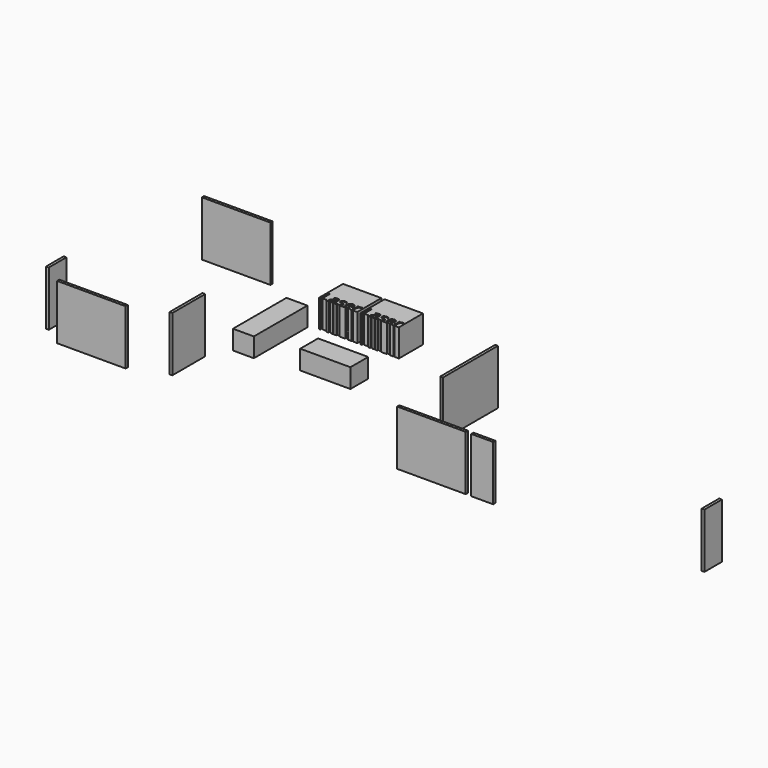
from build123d import *

# Parameters (mm, degrees)
F0_W     = 2479.91771698
F0_H     = 100
F0_W_2   = 20.08228302
F1_DEPTH = 2000
F0_W_3   = 100
F0_H_2   = 800
F0_W_4   = 2500
F0_W_5   = 800
F0_H_3   = 1500
F0_H_4   = 2500
F0_W_6   = 1828.8
F0_H_5   = 812.8
F4_DEPTH = 700
F0_W_7   = 762
F0_H_6   = 2438.4
F5_DEPTH = 1000


# Not quite as in the source:
# - the program builds the solid bodies; features that only make, move or delete a surface that nothing else refers to are left out


with BuildPart() as f1:
    # F0 (on Top) → F1 (new body)
    with BuildSketch(Plane.XY):
        with Locations((-9960.04114151, 3300)):
            Rectangle(F0_W, F0_H)
        with Locations((-8710.04114151, 3300)):
            Rectangle(F0_W_2, F0_H)
    extrude(amount=F1_DEPTH)


with BuildPart() as f1b:
    # F0 (on Top) → F1, piece 2 (new body)
    with BuildSketch(Plane.XY):
        with Locations((-11950, -2450)):
            Rectangle(F0_W_3, F0_H_2)
    extrude(amount=F1_DEPTH)


with BuildPart() as f1c:
    # F0 (on Top) → F1, piece 3 (new body)
    with BuildSketch(Plane.XY):
        with Locations((-9950, -3300)):
            Rectangle(F0_W_4, F0_H)
    extrude(amount=F1_DEPTH)


with BuildPart() as f1d:
    # F0 (on Top) → F1, piece 4 (new body)
    with BuildSketch(Plane.XY):
        with Locations((4300, -3300)):
            Rectangle(F0_W_5, F0_H)
    extrude(amount=F1_DEPTH)


with BuildPart() as f1e:
    # F0 (on Top) → F1, piece 5 (new body)
    with BuildSketch(Plane.XY):
        with Locations((2450, -3300)):
            Rectangle(F0_W_4, F0_H)
    extrude(amount=F1_DEPTH)


with BuildPart() as f1f:
    # F0 (on Top) → F1, piece 6 (new body)
    with BuildSketch(Plane.XY):
        with Locations((11950, -2450)):
            Rectangle(F0_W_3, F0_H_2)
    extrude(amount=F1_DEPTH)


with BuildPart() as f1g:
    # F0 (on Top) → F1, piece 7 (new body)
    with BuildSketch(Plane.XY):
        with Locations((-7450, -2100)):
            Rectangle(F0_W_3, F0_H_3)
    extrude(amount=F1_DEPTH)


with BuildPart() as f1h:
    # F0 (on Top) → F1, piece 8 (new body)
    with BuildSketch(Plane.XY):
        with Locations((1050, 115.6229972839)):
            Rectangle(F0_W_3, F0_H_4)
    extrude(amount=F1_DEPTH)


with BuildPart() as f4:
    # F0 (on Top) → F4 (new body)
    with BuildSketch(Plane.XY):
        with Locations((-3828.3553308487, 67.7179724663)):
            Rectangle(F0_W_6, F0_H_5)
    extrude(amount=F4_DEPTH)


with BuildPart() as f4b:
    # F0 (on Top) → F4, piece 2 (new body)
    with BuildSketch(Plane.XY):
        with Locations((-6626.9812164307, 645.5204336166)):
            Rectangle(F0_W_7, F0_H_6)
    extrude(amount=F4_DEPTH)


with BuildPart() as f5:
    # F0 (on Top) → F5 (new body)
    with BuildSketch(Plane.XY):
        with BuildLine():
            Line((-4528.5587310791, 3091.9769287109), (-5928.5587310791, 3091.9769287109))
            Line((-5928.5587310791, 3091.9769287109), (-5928.5587310791, 1991.9769287109))
            Line((-5928.5587310791, 1991.9769287109), (-5875.150882701, 1991.9769287109))
            Line((-5875.150882701, 1991.9769287109), (-5875.150882701, 2380.5445389649))
            Line((-5875.150882701, 2380.5445389649), (-5829.9923357444, 2380.5445389649))
            Line((-5829.9923357444, 2380.5445389649), (-5829.9923357444, 2032.88325844))
            Line((-5829.9923357444, 2032.88325844), (-5658.5429371294, 2032.88325844))
            Line((-5658.5429371294, 2032.88325844), (-5658.5429371294, 1991.9769287109))
            Line((-5658.5429371294, 1991.9769287109), (-5566.4860231589, 1991.9769287109))
            add(Edge.make_bspline(
                [(-5566.4860231589, 1991.9769287109), (-5583.9119205595, 1997.5660964187), (-5596.4605656071, 2008.9857976212)],
                knots=[0.4894320446, 0.4894320446, 0.4894320446, 1, 1, 1], degree=2))
            add(Edge.make_bspline(
                [(-5596.4605656071, 2008.9857976212), (-5621.0383811824, 2031.3524602381), (-5621.0383811824, 2072.5139230008)],
                knots=[0, 0, 0, 1, 1, 1], degree=2))
            add(Edge.make_bspline(
                [(-5621.0383811824, 2072.5139230008), (-5621.0383811824, 2160.7049083003), (-5479.9498135721, 2164.9571255278)],
                knots=[0, 0, 0, 1, 1, 1], degree=2))
            Line((-5479.9498135721, 2164.9571255278), (-5430.5390493879, 2166.5729680743))
            Line((-5430.5390493879, 2166.5729680743), (-5430.5390493879, 2184.6874134637))
            add(Edge.make_bspline(
                [(-5430.5390493879, 2184.6874134637), (-5430.5390493879, 2218.9602843178), (-5445.2517209953, 2235.2887984716)],
                knots=[0, 0, 0, 1, 1, 1], degree=2))
            add(Edge.make_bspline(
                [(-5445.2517209953, 2235.2887984716), (-5459.9643926026, 2251.6173126254), (-5492.4513322211, 2251.6173126254)],
                knots=[0, 0, 0, 1, 1, 1], degree=2))
            add(Edge.make_bspline(
                [(-5492.4513322211, 2251.6173126254), (-5528.850311689, 2251.6173126254), (-5574.7742577466, 2229.335694353)],
                knots=[0, 0, 0, 1, 1, 1], degree=2))
            Line((-5574.7742577466, 2229.335694353), (-5588.3813528748, 2263.0982991398))
            add(Edge.make_bspline(
                [(-5588.3813528748, 2263.0982991398), (-5566.8651337033, 2274.7493743433), (-5541.2242638212, 2281.3828332183)],
                knots=[0, 0, 0, 1, 1, 1], degree=2))
            add(Edge.make_bspline(
                [(-5541.2242638212, 2281.3828332183), (-5515.583393939, 2288.0162920933), (-5489.7299131955, 2288.0162920933)],
                knots=[0, 0, 0, 1, 1, 1], degree=2))
            add(Edge.make_bspline(
                [(-5489.7299131955, 2288.0162920933), (-5437.6827743302, 2288.0162920933), (-5412.5521705154, 2264.9267525477)],
                knots=[0, 0, 0, 1, 1, 1], degree=2))
            add(Edge.make_bspline(
                [(-5412.5521705154, 2264.9267525477), (-5387.4215667005, 2241.837213002), (-5387.4215667005, 2190.8106062714)],
                knots=[0, 0, 0, 1, 1, 1], degree=2))
            Line((-5387.4215667005, 2190.8106062714), (-5387.4215667005, 1991.9769287109))
            Line((-5387.4215667005, 1991.9769287109), (-5279.165564816, 1991.9769287109))
            add(Edge.make_bspline(
                [(-5279.165564816, 1991.9769287109), (-5299.4656029078, 1996.5398412124), (-5314.3684747311, 2004.9887134273)],
                knots=[0.5400617249, 0.5400617249, 0.5400617249, 1, 1, 1], degree=2))
            Line((-5314.3684747311, 2004.9887134273), (-5314.3684747311, 2045.8950431563))
            add(Edge.make_bspline(
                [(-5314.3684747311, 2045.8950431563), (-5293.362521627, 2035.2645000874), (-5269.3374942913, 2029.183829452)],
                knots=[0, 0, 0, 1, 1, 1], degree=2))
            add(Edge.make_bspline(
                [(-5269.3374942913, 2029.183829452), (-5245.3124669557, 2023.1031588166), (-5222.9458043387, 2023.1031588166)],
                knots=[0, 0, 0, 1, 1, 1], degree=2))
            add(Edge.make_bspline(
                [(-5222.9458043387, 2023.1031588166), (-5188.417800451, 2023.1031588166), (-5169.8356111666, 2034.116401436)],
                knots=[0, 0, 0, 1, 1, 1], degree=2))
            add(Edge.make_bspline(
                [(-5169.8356111666, 2034.116401436), (-5151.2534218822, 2045.1296440554), (-5151.2534218822, 2067.751439706)],
                knots=[0, 0, 0, 1, 1, 1], degree=2))
            add(Edge.make_bspline(
                [(-5151.2534218822, 2067.751439706), (-5151.2534218822, 2084.7603086162), (-5165.9660934895, 2096.8366055424)],
                knots=[0, 0, 0, 1, 1, 1], degree=2))
            add(Edge.make_bspline(
                [(-5165.9660934895, 2096.8366055424), (-5180.6787650968, 2108.9129024687), (-5223.5411147506, 2125.4115053116)],
                knots=[0, 0, 0, 1, 1, 1], degree=2))
            add(Edge.make_bspline(
                [(-5223.5411147506, 2125.4115053116), (-5264.192311446, 2140.5493986417), (-5281.3287468731, 2151.860296467)],
                knots=[0, 0, 0, 1, 1, 1], degree=2))
            add(Edge.make_bspline(
                [(-5281.3287468731, 2151.860296467), (-5298.4651823001, 2163.1711942923), (-5306.8420502384, 2177.5011663491)],
                knots=[0, 0, 0, 1, 1, 1], degree=2))
            add(Edge.make_bspline(
                [(-5306.8420502384, 2177.5011663491), (-5315.2189181767, 2191.831138406), (-5315.2189181767, 2211.7315150309)],
                knots=[0, 0, 0, 1, 1, 1], degree=2))
            add(Edge.make_bspline(
                [(-5315.2189181767, 2211.7315150309), (-5315.2189181767, 2247.3650953979), (-5286.2187966847, 2267.9883489515)],
                knots=[0, 0, 0, 1, 1, 1], degree=2))
            add(Edge.make_bspline(
                [(-5286.2187966847, 2267.9883489515), (-5257.2186751928, 2288.6116025051), (-5206.787378874, 2288.6116025051)],
                knots=[0, 0, 0, 1, 1, 1], degree=2))
            add(Edge.make_bspline(
                [(-5206.787378874, 2288.6116025051), (-5159.7578563373, 2288.6116025051), (-5114.7693980697, 2269.4766249811)],
                knots=[0, 0, 0, 1, 1, 1], degree=2))
            Line((-5114.7693980697, 2269.4766249811), (-5130.5026018117, 2233.5879115806))
            add(Edge.make_bspline(
                [(-5130.5026018117, 2233.5879115806), (-5174.3004392555, 2251.6173126254), (-5209.9340196224, 2251.6173126254)],
                knots=[0, 0, 0, 1, 1, 1], degree=2))
            add(Edge.make_bspline(
                [(-5209.9340196224, 2251.6173126254), (-5241.3153827618, 2251.6173126254), (-5257.2611973651, 2241.7946908298)],
                knots=[0, 0, 0, 1, 1, 1], degree=2))
            add(Edge.make_bspline(
                [(-5257.2611973651, 2241.7946908298), (-5273.2070119684, 2231.9720690341), (-5273.2070119684, 2214.7080670902)],
                knots=[0, 0, 0, 1, 1, 1], degree=2))
            add(Edge.make_bspline(
                [(-5273.2070119684, 2214.7080670902), (-5273.2070119684, 2202.9719475422), (-5267.2113856776, 2194.765168293)],
                knots=[0, 0, 0, 1, 1, 1], degree=2))
            add(Edge.make_bspline(
                [(-5267.2113856776, 2194.765168293), (-5261.2157593867, 2186.5583890438), (-5247.9488416367, 2179.1170088956)],
                knots=[0, 0, 0, 1, 1, 1], degree=2))
            add(Edge.make_bspline(
                [(-5247.9488416367, 2179.1170088956), (-5234.6819238868, 2171.6756287474), (-5196.9222349061, 2157.5582675519)],
                knots=[0, 0, 0, 1, 1, 1], degree=2))
            add(Edge.make_bspline(
                [(-5196.9222349061, 2157.5582675519), (-5145.1302290745, 2138.6784230616), (-5126.9307393406, 2119.5434455376)],
                knots=[0, 0, 0, 1, 1, 1], degree=2))
            add(Edge.make_bspline(
                [(-5126.9307393406, 2119.5434455376), (-5108.7312496066, 2100.4084680136), (-5108.7312496066, 2071.4083465217)],
                knots=[0, 0, 0, 1, 1, 1], degree=2))
            add(Edge.make_bspline(
                [(-5108.7312496066, 2071.4083465217), (-5108.7312496066, 2030.7571498262), (-5139.0070362668, 2008.6881424152)],
                knots=[0, 0, 0, 1, 1, 1], degree=2))
            add(Edge.make_bspline(
                [(-5139.0070362668, 2008.6881424152), (-5154.3652891477, 1997.4930114529), (-5176.0263007473, 1991.9769287109)],
                knots=[0, 0, 0, 0.5072784088, 0.5072784088, 0.5072784088], degree=2))
            Line((-5176.0263007473, 1991.9769287109), (-4957.8182645501, 1991.9769287109))
            add(Edge.make_bspline(
                [(-4957.8182645501, 1991.9769287109), (-4992.2307684042, 2001.143802815), (-5015.8203031846, 2025.9946665314)],
                knots=[0.3688754729, 0.3688754729, 0.3688754729, 1, 1, 1], degree=2))
            add(Edge.make_bspline(
                [(-5015.8203031846, 2025.9946665314), (-5053.1972926148, 2065.3701980585), (-5053.1972926148, 2135.191604935)],
                knots=[0, 0, 0, 1, 1, 1], degree=2))
            add(Edge.make_bspline(
                [(-5053.1972926148, 2135.191604935), (-5053.1972926148, 2205.6933665678), (-5018.4992000379, 2247.1524845365)],
                knots=[0, 0, 0, 1, 1, 1], degree=2))
            add(Edge.make_bspline(
                [(-5018.4992000379, 2247.1524845365), (-4983.8011074611, 2288.6116025051), (-4925.2905984099, 2288.6116025051)],
                knots=[0, 0, 0, 1, 1, 1], degree=2))
            add(Edge.make_bspline(
                [(-4925.2905984099, 2288.6116025051), (-4870.6070848636, 2288.6116025051), (-4838.7154556569, 2252.5953225877)],
                knots=[0, 0, 0, 1, 1, 1], degree=2))
            add(Edge.make_bspline(
                [(-4838.7154556569, 2252.5953225877), (-4806.8238264503, 2216.5790426704), (-4806.8238264503, 2157.5582675519)],
                knots=[0, 0, 0, 1, 1, 1], degree=2))
            Line((-4806.8238264503, 2157.5582675519), (-4806.8238264503, 2129.6637225391))
            Line((-4806.8238264503, 2129.6637225391), (-5007.4434352463, 2129.6637225391))
            add(Edge.make_bspline(
                [(-5007.4434352463, 2129.6637225391), (-5006.0827257335, 2078.3819827748), (-4981.5049101582, 2051.8056251026)],
                knots=[0, 0, 0, 1, 1, 1], degree=2))
            add(Edge.make_bspline(
                [(-4981.5049101582, 2051.8056251026), (-4956.9270945829, 2025.2292674304), (-4912.2788136936, 2025.2292674304)],
                knots=[0, 0, 0, 1, 1, 1], degree=2))
            add(Edge.make_bspline(
                [(-4912.2788136936, 2025.2292674304), (-4865.2492911569, 2025.2292674304), (-4819.3253450993, 2044.8745110217)],
                knots=[0, 0, 0, 1, 1, 1], degree=2))
            Line((-4819.3253450993, 2044.8745110217), (-4819.3253450993, 2005.4989794946))
            add(Edge.make_bspline(
                [(-4819.3253450993, 2005.4989794946), (-4840.385796796, 1996.4621311301), (-4859.3773185177, 1991.9769287109)],
                knots=[0, 0, 0, 0.9005120931, 0.9005120931, 0.9005120931], degree=2))
            Line((-4859.3773185177, 1991.9769287109), (-4731.5595815225, 1991.9769287109))
            Line((-4731.5595815225, 1991.9769287109), (-4731.5595815225, 2283.2538087984))
            Line((-4731.5595815225, 2283.2538087984), (-4695.1606020547, 2283.2538087984))
            Line((-4695.1606020547, 2283.2538087984), (-4690.0579413816, 2229.335694353))
            Line((-4690.0579413816, 2229.335694353), (-4687.9318327678, 2229.335694353))
            add(Edge.make_bspline(
                [(-4687.9318327678, 2229.335694353), (-4671.7734073031, 2257.7405054331), (-4648.8964786189, 2273.1760539691)],
                knots=[0, 0, 0, 1, 1, 1], degree=2))
            add(Edge.make_bspline(
                [(-4648.8964786189, 2273.1760539691), (-4626.0195499346, 2288.6116025051), (-4598.6352709892, 2288.6116025051)],
                knots=[0, 0, 0, 1, 1, 1], degree=2))
            add(Edge.make_bspline(
                [(-4598.6352709892, 2288.6116025051), (-4579.2451604315, 2288.6116025051), (-4563.8521340678, 2285.3799174122)],
                knots=[0, 0, 0, 1, 1, 1], degree=2))
            Line((-4563.8521340678, 2285.3799174122), (-4569.9753268755, 2244.4735876831))
            add(Edge.make_bspline(
                [(-4569.9753268755, 2244.4735876831), (-4588.0047279203, 2248.470671877), (-4601.8669560821, 2248.470671877)],
                knots=[0, 0, 0, 1, 1, 1], degree=2))
            add(Edge.make_bspline(
                [(-4601.8669560821, 2248.470671877), (-4637.2454034154, 2248.470671877), (-4662.333485058, 2219.768205591)],
                knots=[0, 0, 0, 1, 1, 1], degree=2))
            add(Edge.make_bspline(
                [(-4662.333485058, 2219.768205591), (-4687.4215667005, 2191.065739305), (-4687.4215667005, 2148.2884339958)],
                knots=[0, 0, 0, 1, 1, 1], degree=2))
            Line((-4687.4215667005, 2148.2884339958), (-4687.4215667005, 1991.9769287109))
            Line((-4687.4215667005, 1991.9769287109), (-4528.5587310791, 1991.9769287109))
            Line((-4528.5587310791, 1991.9769287109), (-4528.5587310791, 3091.9769287109))
        make_face()
    extrude(amount=F5_DEPTH)


with BuildPart() as f5b:
    # F0 (on Top) → F5, piece 2 (new body)
    with BuildSketch(Plane.XY):
        with BuildLine():
            add(Edge.make_bspline(
                [(-4872.6906713051, 2229.4207386976), (-4891.2728605895, 2251.6173126254), (-4925.8859088218, 2251.6173126254)],
                knots=[0, 0, 0, 1, 1, 1], degree=2))
            add(Edge.make_bspline(
                [(-4925.8859088218, 2251.6173126254), (-4960.9241787768, 2251.6173126254), (-4981.8025653641, 2228.7829061134)],
                knots=[0, 0, 0, 1, 1, 1], degree=2))
            add(Edge.make_bspline(
                [(-4981.8025653641, 2228.7829061134), (-5002.6809519514, 2205.9484996015), (-5006.4229031117, 2165.5524359397)],
                knots=[0, 0, 0, 1, 1, 1], degree=2))
            Line((-5006.4229031117, 2165.5524359397), (-4854.1084820207, 2165.5524359397))
            add(Edge.make_bspline(
                [(-4854.1084820207, 2165.5524359397), (-4854.1084820207, 2207.2241647697), (-4872.6906713051, 2229.4207386976)],
                knots=[0, 0, 0, 1, 1, 1], degree=2))
        make_face()
    extrude(amount=F5_DEPTH)


with BuildPart() as f5c:
    # F0 (on Top) → F5, piece 3 (new body)
    with BuildSketch(Plane.XY):
        with BuildLine():
            add(Edge.make_bspline(
                [(-5560.3167191729, 2035.5621552934), (-5545.8591805992, 2023.1031588166), (-5519.8356111666, 2023.1031588166)],
                knots=[0, 0, 0, 1, 1, 1], degree=2))
            add(Edge.make_bspline(
                [(-5519.8356111666, 2023.1031588166), (-5478.5891040593, 2023.1031588166), (-5455.0743427909, 2045.6824322949)],
                knots=[0, 0, 0, 1, 1, 1], degree=2))
            add(Edge.make_bspline(
                [(-5455.0743427909, 2045.6824322949), (-5431.5595815225, 2068.2617057733), (-5431.5595815225, 2108.9129024687)],
                knots=[0, 0, 0, 1, 1, 1], degree=2))
            Line((-5431.5595815225, 2108.9129024687), (-5431.5595815225, 2135.191604935))
            Line((-5431.5595815225, 2135.191604935), (-5475.6975963446, 2133.4056736994))
            add(Edge.make_bspline(
                [(-5475.6975963446, 2133.4056736994), (-5528.3400456217, 2131.5346981193), (-5551.5571516841, 2117.0346373733)],
                knots=[0, 0, 0, 1, 1, 1], degree=2))
            add(Edge.make_bspline(
                [(-5551.5571516841, 2117.0346373733), (-5574.7742577466, 2102.5345766274), (-5574.7742577466, 2072.0036569335)],
                knots=[0, 0, 0, 1, 1, 1], degree=2))
            add(Edge.make_bspline(
                [(-5574.7742577466, 2072.0036569335), (-5574.7742577466, 2048.0211517701), (-5560.3167191729, 2035.5621552934)],
                knots=[0, 0, 0, 1, 1, 1], degree=2))
        make_face()
    extrude(amount=F5_DEPTH)


with BuildPart() as f5d:
    # F0 (on Top) → F5, piece 4 (new body)
    with BuildSketch(Plane.XY):
        with BuildLine():
            add(Edge.make_bspline(
                [(-5474.4644533486, 1996.3567124553), (-5480.0535922073, 1993.8421490002), (-5486.3657987835, 1991.9769287109)],
                knots=[0, 0, 0, 0.2582329607, 0.2582329607, 0.2582329607], degree=2))
            Line((-5486.3657987835, 1991.9769287109), (-5420.1636393527, 1991.9769287109))
            Line((-5420.1636393527, 1991.9769287109), (-5428.9232068415, 2033.4785688519))
            Line((-5428.9232068415, 2033.4785688519), (-5431.0493154552, 2033.4785688519))
            add(Edge.make_bspline(
                [(-5431.0493154552, 2033.4785688519), (-5452.8206676603, 2006.0942899064), (-5474.4644533486, 1996.3567124553)],
                knots=[0, 0, 0, 1, 1, 1], degree=2))
        make_face()
    extrude(amount=F5_DEPTH)


with BuildPart() as f5e:
    # F0 (on Top) → F5, piece 5 (new body)
    with BuildSketch(Plane.XY):
        with BuildLine():
            Line((-3012.7561569214, 3091.9769287109), (-4412.7561569214, 3091.9769287109))
            Line((-4412.7561569214, 3091.9769287109), (-4412.7561569214, 1991.9769287109))
            Line((-4412.7561569214, 1991.9769287109), (-4359.3483085433, 1991.9769287109))
            Line((-4359.3483085433, 1991.9769287109), (-4359.3483085433, 2380.5445389649))
            Line((-4359.3483085433, 2380.5445389649), (-4314.1897615867, 2380.5445389649))
            Line((-4314.1897615867, 2380.5445389649), (-4314.1897615867, 2032.88325844))
            Line((-4314.1897615867, 2032.88325844), (-4142.7403629717, 2032.88325844))
            Line((-4142.7403629717, 2032.88325844), (-4142.7403629717, 1991.9769287109))
            Line((-4142.7403629717, 1991.9769287109), (-4050.6834490011, 1991.9769287109))
            add(Edge.make_bspline(
                [(-4050.6834490011, 1991.9769287109), (-4068.1093464018, 1997.5660964187), (-4080.6579914494, 2008.9857976212)],
                knots=[0.4894320446, 0.4894320446, 0.4894320446, 1, 1, 1], degree=2))
            add(Edge.make_bspline(
                [(-4080.6579914494, 2008.9857976212), (-4105.2358070247, 2031.3524602381), (-4105.2358070247, 2072.5139230008)],
                knots=[0, 0, 0, 1, 1, 1], degree=2))
            add(Edge.make_bspline(
                [(-4105.2358070247, 2072.5139230008), (-4105.2358070247, 2160.7049083003), (-3964.1472394144, 2164.9571255278)],
                knots=[0, 0, 0, 1, 1, 1], degree=2))
            Line((-3964.1472394144, 2164.9571255278), (-3914.7364752302, 2166.5729680743))
            Line((-3914.7364752302, 2166.5729680743), (-3914.7364752302, 2184.6874134637))
            add(Edge.make_bspline(
                [(-3914.7364752302, 2184.6874134637), (-3914.7364752302, 2218.9602843178), (-3929.4491468376, 2235.2887984716)],
                knots=[0, 0, 0, 1, 1, 1], degree=2))
            add(Edge.make_bspline(
                [(-3929.4491468376, 2235.2887984716), (-3944.1618184449, 2251.6173126254), (-3976.6487580634, 2251.6173126254)],
                knots=[0, 0, 0, 1, 1, 1], degree=2))
            add(Edge.make_bspline(
                [(-3976.6487580634, 2251.6173126254), (-4013.0477375313, 2251.6173126254), (-4058.9716835889, 2229.335694353)],
                knots=[0, 0, 0, 1, 1, 1], degree=2))
            Line((-4058.9716835889, 2229.335694353), (-4072.578778717, 2263.0982991398))
            add(Edge.make_bspline(
                [(-4072.578778717, 2263.0982991398), (-4051.0625595456, 2274.7493743433), (-4025.4216896635, 2281.3828332183)],
                knots=[0, 0, 0, 1, 1, 1], degree=2))
            add(Edge.make_bspline(
                [(-4025.4216896635, 2281.3828332183), (-3999.7808197813, 2288.0162920933), (-3973.9273390378, 2288.0162920933)],
                knots=[0, 0, 0, 1, 1, 1], degree=2))
            add(Edge.make_bspline(
                [(-3973.9273390378, 2288.0162920933), (-3921.8802001725, 2288.0162920933), (-3896.7495963577, 2264.9267525477)],
                knots=[0, 0, 0, 1, 1, 1], degree=2))
            add(Edge.make_bspline(
                [(-3896.7495963577, 2264.9267525477), (-3871.6189925428, 2241.837213002), (-3871.6189925428, 2190.8106062714)],
                knots=[0, 0, 0, 1, 1, 1], degree=2))
            Line((-3871.6189925428, 2190.8106062714), (-3871.6189925428, 1991.9769287109))
            Line((-3871.6189925428, 1991.9769287109), (-3763.3629906583, 1991.9769287109))
            add(Edge.make_bspline(
                [(-3763.3629906583, 1991.9769287109), (-3783.6630287501, 1996.5398412124), (-3798.5659005734, 2004.9887134273)],
                knots=[0.5400617249, 0.5400617249, 0.5400617249, 1, 1, 1], degree=2))
            Line((-3798.5659005734, 2004.9887134273), (-3798.5659005734, 2045.8950431563))
            add(Edge.make_bspline(
                [(-3798.5659005734, 2045.8950431563), (-3777.5599474693, 2035.2645000874), (-3753.5349201336, 2029.183829452)],
                knots=[0, 0, 0, 1, 1, 1], degree=2))
            add(Edge.make_bspline(
                [(-3753.5349201336, 2029.183829452), (-3729.5098927979, 2023.1031588166), (-3707.143230181, 2023.1031588166)],
                knots=[0, 0, 0, 1, 1, 1], degree=2))
            add(Edge.make_bspline(
                [(-3707.143230181, 2023.1031588166), (-3672.6152262933, 2023.1031588166), (-3654.0330370089, 2034.116401436)],
                knots=[0, 0, 0, 1, 1, 1], degree=2))
            add(Edge.make_bspline(
                [(-3654.0330370089, 2034.116401436), (-3635.4508477244, 2045.1296440554), (-3635.4508477244, 2067.751439706)],
                knots=[0, 0, 0, 1, 1, 1], degree=2))
            add(Edge.make_bspline(
                [(-3635.4508477244, 2067.751439706), (-3635.4508477244, 2084.7603086162), (-3650.1635193318, 2096.8366055424)],
                knots=[0, 0, 0, 1, 1, 1], degree=2))
            add(Edge.make_bspline(
                [(-3650.1635193318, 2096.8366055424), (-3664.8761909391, 2108.9129024687), (-3707.7385405929, 2125.4115053116)],
                knots=[0, 0, 0, 1, 1, 1], degree=2))
            add(Edge.make_bspline(
                [(-3707.7385405929, 2125.4115053116), (-3748.3897372883, 2140.5493986417), (-3765.5261727153, 2151.860296467)],
                knots=[0, 0, 0, 1, 1, 1], degree=2))
            add(Edge.make_bspline(
                [(-3765.5261727153, 2151.860296467), (-3782.6626081424, 2163.1711942923), (-3791.0394760807, 2177.5011663491)],
                knots=[0, 0, 0, 1, 1, 1], degree=2))
            add(Edge.make_bspline(
                [(-3791.0394760807, 2177.5011663491), (-3799.4163440189, 2191.831138406), (-3799.4163440189, 2211.7315150309)],
                knots=[0, 0, 0, 1, 1, 1], degree=2))
            add(Edge.make_bspline(
                [(-3799.4163440189, 2211.7315150309), (-3799.4163440189, 2247.3650953979), (-3770.416222527, 2267.9883489515)],
                knots=[0, 0, 0, 1, 1, 1], degree=2))
            add(Edge.make_bspline(
                [(-3770.416222527, 2267.9883489515), (-3741.4161010351, 2288.6116025051), (-3690.9848047163, 2288.6116025051)],
                knots=[0, 0, 0, 1, 1, 1], degree=2))
            add(Edge.make_bspline(
                [(-3690.9848047163, 2288.6116025051), (-3643.9552821796, 2288.6116025051), (-3598.966823912, 2269.4766249811)],
                knots=[0, 0, 0, 1, 1, 1], degree=2))
            Line((-3598.966823912, 2269.4766249811), (-3614.700027654, 2233.5879115806))
            add(Edge.make_bspline(
                [(-3614.700027654, 2233.5879115806), (-3658.4978650978, 2251.6173126254), (-3694.1314454647, 2251.6173126254)],
                knots=[0, 0, 0, 1, 1, 1], degree=2))
            add(Edge.make_bspline(
                [(-3694.1314454647, 2251.6173126254), (-3725.512808604, 2251.6173126254), (-3741.4586232074, 2241.7946908298)],
                knots=[0, 0, 0, 1, 1, 1], degree=2))
            add(Edge.make_bspline(
                [(-3741.4586232074, 2241.7946908298), (-3757.4044378107, 2231.9720690341), (-3757.4044378107, 2214.7080670902)],
                knots=[0, 0, 0, 1, 1, 1], degree=2))
            add(Edge.make_bspline(
                [(-3757.4044378107, 2214.7080670902), (-3757.4044378107, 2202.9719475422), (-3751.4088115199, 2194.765168293)],
                knots=[0, 0, 0, 1, 1, 1], degree=2))
            add(Edge.make_bspline(
                [(-3751.4088115199, 2194.765168293), (-3745.413185229, 2186.5583890438), (-3732.146267479, 2179.1170088956)],
                knots=[0, 0, 0, 1, 1, 1], degree=2))
            add(Edge.make_bspline(
                [(-3732.146267479, 2179.1170088956), (-3718.8793497291, 2171.6756287474), (-3681.1196607484, 2157.5582675519)],
                knots=[0, 0, 0, 1, 1, 1], degree=2))
            add(Edge.make_bspline(
                [(-3681.1196607484, 2157.5582675519), (-3629.3276549168, 2138.6784230616), (-3611.1281651828, 2119.5434455376)],
                knots=[0, 0, 0, 1, 1, 1], degree=2))
            add(Edge.make_bspline(
                [(-3611.1281651828, 2119.5434455376), (-3592.9286754489, 2100.4084680136), (-3592.9286754489, 2071.4083465217)],
                knots=[0, 0, 0, 1, 1, 1], degree=2))
            add(Edge.make_bspline(
                [(-3592.9286754489, 2071.4083465217), (-3592.9286754489, 2030.7571498262), (-3623.2044621091, 2008.6881424152)],
                knots=[0, 0, 0, 1, 1, 1], degree=2))
            add(Edge.make_bspline(
                [(-3623.2044621091, 2008.6881424152), (-3638.56271499, 1997.4930114529), (-3660.2237265896, 1991.9769287109)],
                knots=[0, 0, 0, 0.5072784088, 0.5072784088, 0.5072784088], degree=2))
            Line((-3660.2237265896, 1991.9769287109), (-3442.0156903924, 1991.9769287109))
            add(Edge.make_bspline(
                [(-3442.0156903924, 1991.9769287109), (-3476.4281942464, 2001.143802815), (-3500.0177290268, 2025.9946665314)],
                knots=[0.3688754729, 0.3688754729, 0.3688754729, 1, 1, 1], degree=2))
            add(Edge.make_bspline(
                [(-3500.0177290268, 2025.9946665314), (-3537.394718457, 2065.3701980585), (-3537.394718457, 2135.191604935)],
                knots=[0, 0, 0, 1, 1, 1], degree=2))
            add(Edge.make_bspline(
                [(-3537.394718457, 2135.191604935), (-3537.394718457, 2205.6933665678), (-3502.6966258802, 2247.1524845365)],
                knots=[0, 0, 0, 1, 1, 1], degree=2))
            add(Edge.make_bspline(
                [(-3502.6966258802, 2247.1524845365), (-3467.9985333034, 2288.6116025051), (-3409.4880242522, 2288.6116025051)],
                knots=[0, 0, 0, 1, 1, 1], degree=2))
            add(Edge.make_bspline(
                [(-3409.4880242522, 2288.6116025051), (-3354.8045107059, 2288.6116025051), (-3322.9128814992, 2252.5953225877)],
                knots=[0, 0, 0, 1, 1, 1], degree=2))
            add(Edge.make_bspline(
                [(-3322.9128814992, 2252.5953225877), (-3291.0212522925, 2216.5790426704), (-3291.0212522925, 2157.5582675519)],
                knots=[0, 0, 0, 1, 1, 1], degree=2))
            Line((-3291.0212522925, 2157.5582675519), (-3291.0212522925, 2129.6637225391))
            Line((-3291.0212522925, 2129.6637225391), (-3491.6408610886, 2129.6637225391))
            add(Edge.make_bspline(
                [(-3491.6408610886, 2129.6637225391), (-3490.2801515757, 2078.3819827748), (-3465.7023360005, 2051.8056251026)],
                knots=[0, 0, 0, 1, 1, 1], degree=2))
            add(Edge.make_bspline(
                [(-3465.7023360005, 2051.8056251026), (-3441.1245204252, 2025.2292674304), (-3396.4762395359, 2025.2292674304)],
                knots=[0, 0, 0, 1, 1, 1], degree=2))
            add(Edge.make_bspline(
                [(-3396.4762395359, 2025.2292674304), (-3349.4467169991, 2025.2292674304), (-3303.5227709416, 2044.8745110217)],
                knots=[0, 0, 0, 1, 1, 1], degree=2))
            Line((-3303.5227709416, 2044.8745110217), (-3303.5227709416, 2005.4989794946))
            add(Edge.make_bspline(
                [(-3303.5227709416, 2005.4989794946), (-3324.5832226383, 1996.4621311301), (-3343.57474436, 1991.9769287109)],
                knots=[0, 0, 0, 0.9005120931, 0.9005120931, 0.9005120931], degree=2))
            Line((-3343.57474436, 1991.9769287109), (-3215.7570073648, 1991.9769287109))
            Line((-3215.7570073648, 1991.9769287109), (-3215.7570073648, 2283.2538087984))
            Line((-3215.7570073648, 2283.2538087984), (-3179.358027897, 2283.2538087984))
            Line((-3179.358027897, 2283.2538087984), (-3174.2553672239, 2229.335694353))
            Line((-3174.2553672239, 2229.335694353), (-3172.1292586101, 2229.335694353))
            add(Edge.make_bspline(
                [(-3172.1292586101, 2229.335694353), (-3155.9708331454, 2257.7405054331), (-3133.0939044612, 2273.1760539691)],
                knots=[0, 0, 0, 1, 1, 1], degree=2))
            add(Edge.make_bspline(
                [(-3133.0939044612, 2273.1760539691), (-3110.2169757769, 2288.6116025051), (-3082.8326968315, 2288.6116025051)],
                knots=[0, 0, 0, 1, 1, 1], degree=2))
            add(Edge.make_bspline(
                [(-3082.8326968315, 2288.6116025051), (-3063.4425862738, 2288.6116025051), (-3048.0495599101, 2285.3799174122)],
                knots=[0, 0, 0, 1, 1, 1], degree=2))
            Line((-3048.0495599101, 2285.3799174122), (-3054.1727527178, 2244.4735876831))
            add(Edge.make_bspline(
                [(-3054.1727527178, 2244.4735876831), (-3072.2021537626, 2248.470671877), (-3086.0643819244, 2248.470671877)],
                knots=[0, 0, 0, 1, 1, 1], degree=2))
            add(Edge.make_bspline(
                [(-3086.0643819244, 2248.470671877), (-3121.4428292577, 2248.470671877), (-3146.5309109002, 2219.768205591)],
                knots=[0, 0, 0, 1, 1, 1], degree=2))
            add(Edge.make_bspline(
                [(-3146.5309109002, 2219.768205591), (-3171.6189925428, 2191.065739305), (-3171.6189925428, 2148.2884339958)],
                knots=[0, 0, 0, 1, 1, 1], degree=2))
            Line((-3171.6189925428, 2148.2884339958), (-3171.6189925428, 1991.9769287109))
            Line((-3171.6189925428, 1991.9769287109), (-3012.7561569214, 1991.9769287109))
            Line((-3012.7561569214, 1991.9769287109), (-3012.7561569214, 3091.9769287109))
        make_face()
    extrude(amount=F5_DEPTH)


with BuildPart() as f5f:
    # F0 (on Top) → F5, piece 6 (new body)
    with BuildSketch(Plane.XY):
        with BuildLine():
            add(Edge.make_bspline(
                [(-4044.5141450152, 2035.5621552934), (-4030.0566064415, 2023.1031588166), (-4004.0330370089, 2023.1031588166)],
                knots=[0, 0, 0, 1, 1, 1], degree=2))
            add(Edge.make_bspline(
                [(-4004.0330370089, 2023.1031588166), (-3962.7865299016, 2023.1031588166), (-3939.2717686332, 2045.6824322949)],
                knots=[0, 0, 0, 1, 1, 1], degree=2))
            add(Edge.make_bspline(
                [(-3939.2717686332, 2045.6824322949), (-3915.7570073648, 2068.2617057733), (-3915.7570073648, 2108.9129024687)],
                knots=[0, 0, 0, 1, 1, 1], degree=2))
            Line((-3915.7570073648, 2108.9129024687), (-3915.7570073648, 2135.191604935))
            Line((-3915.7570073648, 2135.191604935), (-3959.8950221868, 2133.4056736994))
            add(Edge.make_bspline(
                [(-3959.8950221868, 2133.4056736994), (-4012.537471464, 2131.5346981193), (-4035.7545775264, 2117.0346373733)],
                knots=[0, 0, 0, 1, 1, 1], degree=2))
            add(Edge.make_bspline(
                [(-4035.7545775264, 2117.0346373733), (-4058.9716835889, 2102.5345766274), (-4058.9716835889, 2072.0036569335)],
                knots=[0, 0, 0, 1, 1, 1], degree=2))
            add(Edge.make_bspline(
                [(-4058.9716835889, 2072.0036569335), (-4058.9716835889, 2048.0211517701), (-4044.5141450152, 2035.5621552934)],
                knots=[0, 0, 0, 1, 1, 1], degree=2))
        make_face()
    extrude(amount=F5_DEPTH)


with BuildPart() as f5g:
    # F0 (on Top) → F5, piece 7 (new body)
    with BuildSketch(Plane.XY):
        with BuildLine():
            add(Edge.make_bspline(
                [(-3958.6618791909, 1996.3567124553), (-3964.2510180496, 1993.8421490002), (-3970.5632246258, 1991.9769287109)],
                knots=[0, 0, 0, 0.2582329607, 0.2582329607, 0.2582329607], degree=2))
            Line((-3970.5632246258, 1991.9769287109), (-3904.361065195, 1991.9769287109))
            Line((-3904.361065195, 1991.9769287109), (-3913.1206326837, 2033.4785688519))
            Line((-3913.1206326837, 2033.4785688519), (-3915.2467412975, 2033.4785688519))
            add(Edge.make_bspline(
                [(-3915.2467412975, 2033.4785688519), (-3937.0180935026, 2006.0942899064), (-3958.6618791909, 1996.3567124553)],
                knots=[0, 0, 0, 1, 1, 1], degree=2))
        make_face()
    extrude(amount=F5_DEPTH)


with BuildPart() as f5h:
    # F0 (on Top) → F5, piece 8 (new body)
    with BuildSketch(Plane.XY):
        with BuildLine():
            add(Edge.make_bspline(
                [(-3356.8880971474, 2229.4207386976), (-3375.4702864318, 2251.6173126254), (-3410.0833346641, 2251.6173126254)],
                knots=[0, 0, 0, 1, 1, 1], degree=2))
            add(Edge.make_bspline(
                [(-3410.0833346641, 2251.6173126254), (-3445.1216046191, 2251.6173126254), (-3465.9999912064, 2228.7829061134)],
                knots=[0, 0, 0, 1, 1, 1], degree=2))
            add(Edge.make_bspline(
                [(-3465.9999912064, 2228.7829061134), (-3486.8783777937, 2205.9484996015), (-3490.6203289539, 2165.5524359397)],
                knots=[0, 0, 0, 1, 1, 1], degree=2))
            Line((-3490.6203289539, 2165.5524359397), (-3338.3059078629, 2165.5524359397))
            add(Edge.make_bspline(
                [(-3338.3059078629, 2165.5524359397), (-3338.3059078629, 2207.2241647697), (-3356.8880971474, 2229.4207386976)],
                knots=[0, 0, 0, 1, 1, 1], degree=2))
        make_face()
    extrude(amount=F5_DEPTH)


solid = Compound([f1.part, f1b.part, f1c.part, f1d.part, f1e.part, f1f.part, f1g.part, f1h.part, f4.part, f4b.part, f5.part, f5b.part, f5c.part, f5d.part, f5e.part, f5f.part, f5g.part, f5h.part])
